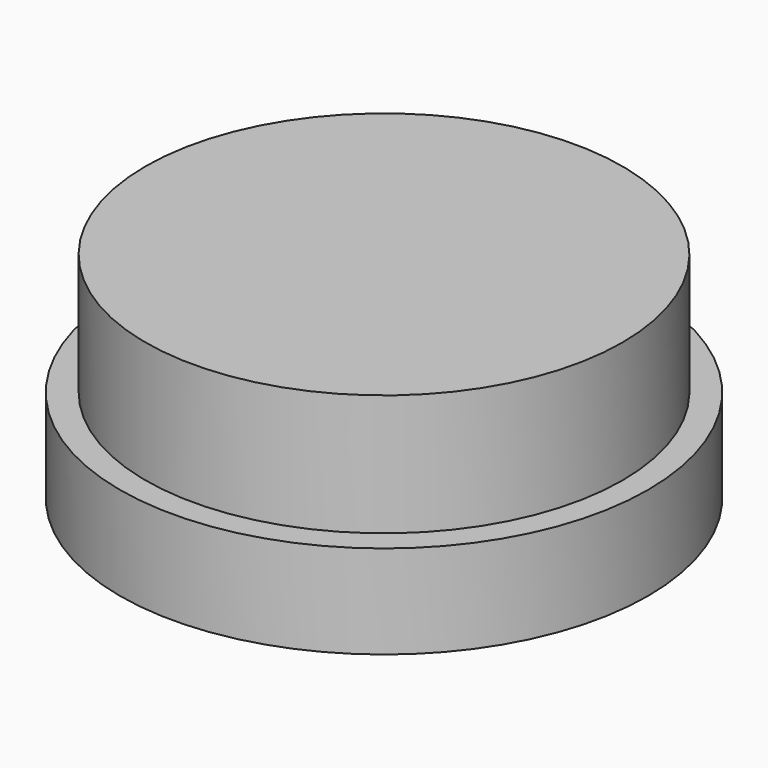
from build123d import *

# Parameters (mm, degrees)
F0_R     = 28.2834401036
F1_DEPTH = 10
F2_R     = 25.5390736026
F3_DEPTH = 13


# Not quite as in the source:
# - a feature of the source that left no trace in its solid (it failed there, or was rolled back) is left out


with BuildPart() as f1:
    # F0 (on Top) → F1 (new body)
    with BuildSketch(Plane.XY):
        Circle(F0_R)
    extrude(amount=F1_DEPTH)

    # F2 (on face) → F3 (join)
    with BuildSketch(Plane.XY.offset(10)):
        Circle(F2_R)
    extrude(amount=F3_DEPTH)


solid = f1.part
